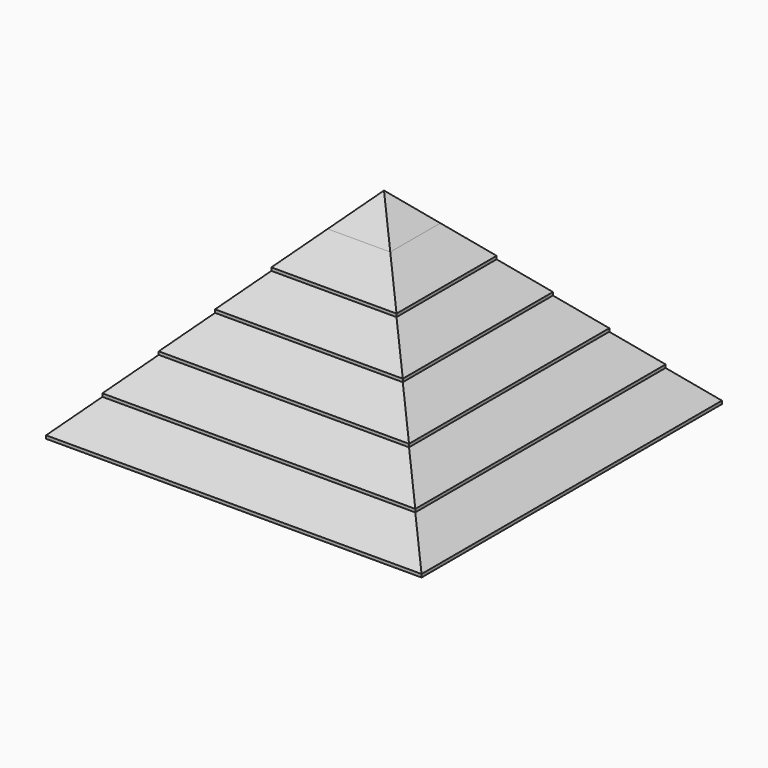
from build123d import *

# Parameters (mm, degrees)
F0_W      = 76.2
F0_H      = 76.2
F1_DEPTH  = 13.97
F2_W      = 63.5
F2_H      = 63.5
F3_DEPTH  = 13.97
F4_W      = 50.8
F4_H      = 50.8
F5_DEPTH  = 13.97
F6_W      = 38.1
F6_H      = 38.1
F7_DEPTH  = 13.97
F8_W      = 25.4
F8_H      = 25.4
F9_DEPTH  = 13.97
F10_SIZE  = 12.69999
F9_FACE_W = 25.40002
F9_FACE_H = 25.40002


# Not quite as in the source:
# - a fillet or chamfer is up to 0.001 mm smaller than in the source, because OpenCascade refuses the exact size


with BuildPart() as f1:
    # F0 (on Top) → F1 (new body)
    with BuildSketch(Plane.XY):
        with Locations((38.1, 38.1)):
            Rectangle(F0_W, F0_H)
        with Locations((38.1, -38.1)):
            Rectangle(F0_W, F0_H)
        with Locations((-38.1, -38.1)):
            Rectangle(F0_W, F0_H)
        with Locations((-38.1, 38.1)):
            Rectangle(F0_W, F0_H)
    extrude(amount=F1_DEPTH)

    # F2 (on face) → F3 (join)
    with BuildSketch(Plane.XY.offset(13.97)):
        with Locations((-31.75, -31.75)):
            Rectangle(F2_W, F2_H)
        with Locations((-31.75, 31.75)):
            Rectangle(F2_W, F2_H)
        with Locations((31.75, 31.75)):
            Rectangle(F2_W, F2_H)
        with Locations((31.75, -31.75)):
            Rectangle(F2_W, F2_H)
    extrude(amount=F3_DEPTH)

    # F4 (on face) → F5 (join)
    with BuildSketch(Plane.XY.offset(27.94)):
        with Locations((-25.4, -25.4)):
            Rectangle(F4_W, F4_H)
        with Locations((-25.4, 25.4)):
            Rectangle(F4_W, F4_H)
        with Locations((25.4, 25.4)):
            Rectangle(F4_W, F4_H)
        with Locations((25.4, -25.4)):
            Rectangle(F4_W, F4_H)
    extrude(amount=F5_DEPTH)

    # F6 (on face) → F7 (join)
    with BuildSketch(Plane.XY.offset(41.91)):
        with Locations((19.05, -19.05)):
            Rectangle(F6_W, F6_H)
        with Locations((-19.05, -19.05)):
            Rectangle(F6_W, F6_H)
        with Locations((19.05, 19.05)):
            Rectangle(F6_W, F6_H)
        with Locations((-19.05, 19.05)):
            Rectangle(F6_W, F6_H)
    extrude(amount=F7_DEPTH)

    # F8 (on face) → F9 (join)
    with BuildSketch(Plane.XY.offset(55.88)):
        with Locations((-12.7, -12.7)):
            Rectangle(F8_W, F8_H)
        with Locations((-12.7, 12.7)):
            Rectangle(F8_W, F8_H)
        with Locations((12.7, 12.7)):
            Rectangle(F8_W, F8_H)
        with Locations((12.7, -12.7)):
            Rectangle(F8_W, F8_H)
    extrude(amount=F9_DEPTH)

    # F10 (size 12.7 in the source; OpenCascade refuses exactly that, so slightly less here)
    f10_edges = [f1.edges().sort_by_distance(p)[0] for p in [
        (-25.4, 0, 69.85),
        (0, -25.4, 69.85),
        (25.4, 0, 69.85),
        (0, 25.4, 69.85),
        (0, 38.1, 55.88),
        (-38.1, 0, 55.88),
        (0, -38.1, 55.88),
        (38.1, 0, 55.88),
        (50.8, 0, 41.91),
        (0, 50.8, 41.91),
        (-50.8, 0, 41.91),
        (0, -50.8, 41.91),
        (-63.5, 0, 27.94),
        (0, 63.5, 27.94),
        (63.5, 0, 27.94),
        (0, -63.5, 27.94),
        (76.2, 0, 13.97),
        (0, 76.2, 13.97),
        (-76.2, 0, 13.97),
        (0, -76.2, 13.97),
    ]]
    chamfer(f10_edges, length=F10_SIZE)

    # F9_face (on face) → F13 section 0
    with BuildSketch(Plane.XY.offset(69.85), mode=Mode.PRIVATE) as f13_s0:
        Rectangle(F9_FACE_W, F9_FACE_H)
    loft([f13_s0.sketch, Vertex(0, 0, 82.55)])


solid = f1.part
